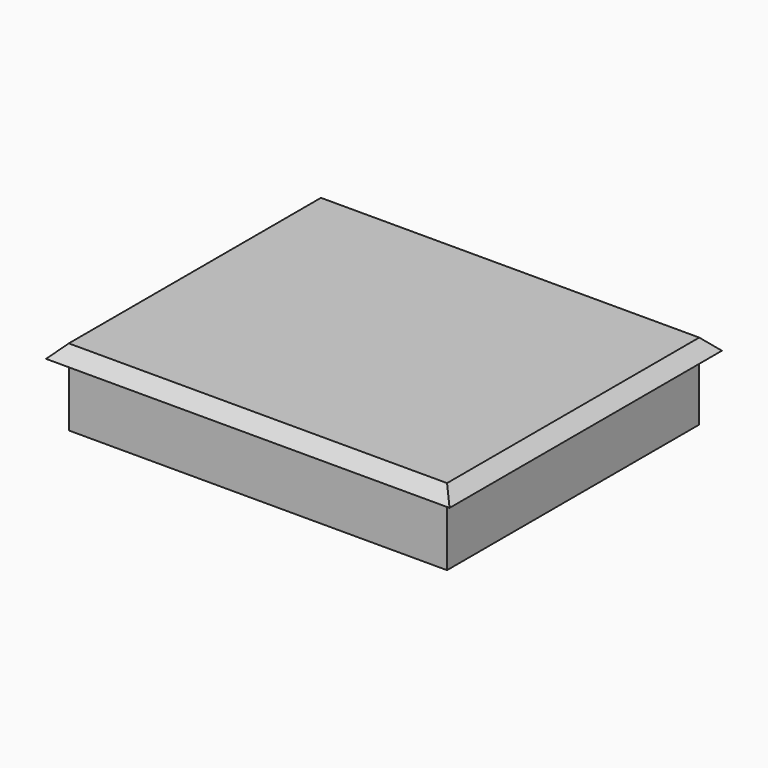
from build123d import *

# Parameters (mm, degrees)
F0_W     = 30000
F0_H     = 25000
F1_DEPTH = 5080
F2_W     = 32000
F2_H     = 27000
F3_DEPTH = 1000
F4_SIZE  = 999.99999


# Not quite as in the source:
# - a fillet or chamfer is up to 0.001 mm smaller than in the source, because OpenCascade refuses the exact size


with BuildPart() as f1:
    # F0 (on Top) → F1 (new body)
    with BuildSketch(Plane.XY):
        with Locations((14.6500738338, 3645.5633971739)):
            Rectangle(F0_W, F0_H)
    extrude(amount=F1_DEPTH)

    # F2 (on face) → F3 (join)
    with BuildSketch(Plane.XY.offset(5080)):
        with Locations((14.6500738338, 3645.5633971739)):
            Rectangle(F2_W, F2_H)
    extrude(amount=F3_DEPTH)

    # F4 (size 1000 in the source; OpenCascade refuses exactly that, so slightly less here)
    f4_edges = [f1.edges().sort_by_distance(p)[0] for p in [
        (14.650074, -9854.436603, 6080),
        (16014.650074, 3645.563397, 6080),
        (14.650074, 17145.563397, 6080),
        (-15985.349926, 3645.563397, 6080),
    ]]
    chamfer(f4_edges, length=F4_SIZE)


solid = f1.part
